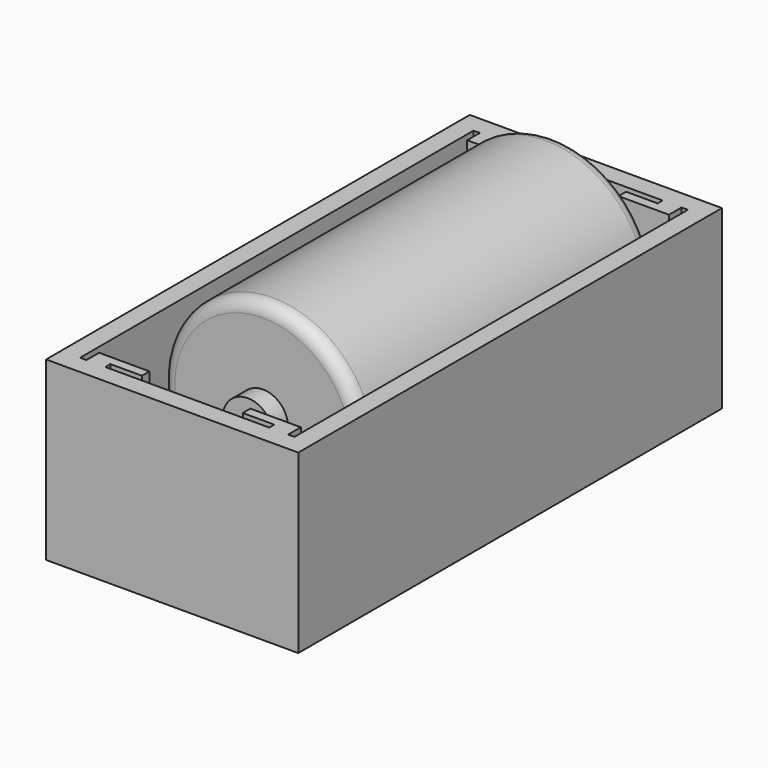
from build123d import *

# Parameters (mm, degrees)
F0_R            = 16
F1_DEPTH        = 58
F2_R            = 4
F3_DEPTH        = 3
F4_R            = 2
F6_W            = 40
F6_H            = 84
F7_DEPTH        = 3
F8_W            = 40
F8_H            = 84
F8_W_2          = 34
F8_H_2          = 78
F9_DEPTH        = 25
F10_R           = 5.8847523539
F11_DEPTH       = 25
F13_DEPTH       = 25
F14_TEXT_SIZE   = 13.9910155364
F14_TEXT_SIZE_2 = 12.9334014168
F15_DEPTH       = 0.5


# Not quite as in the source:
# - Text() gives the source's letters only with a copy of the font that has no kerning and outlines rounded to 1/6400 em; it was checked with that copy


with BuildPart() as f1:
    # F0 (on Front) → F1 (new body)
    with BuildSketch(Plane.XZ):
        Circle(F0_R)
    extrude(amount=F1_DEPTH)

    # F2 (on face) → F3 (join)
    with BuildSketch(Plane.XZ.offset(58)):
        Circle(F2_R)
    extrude(amount=F3_DEPTH)

    # F4
    f4_edges = [f1.edges().sort_by_distance(p)[0] for p in [
        (-16, -58, 0),
        (-16, 0, 0),
    ]]
    fillet(f4_edges, radius=F4_R)


with BuildPart() as f7:
    # F6 (on offset) → F7 (new body)
    with BuildSketch(Plane.XY.offset(-16)):
        with Locations((0, -34)):
            Rectangle(F6_W, F6_H)
    extrude(amount=-F7_DEPTH)

    # F8 (on face) → F9 (join)
    with BuildSketch(Plane.XY.offset(-16)):
        with Locations((0, -34)):
            Rectangle(F8_W, F8_H)
        with Locations((0, -34)):
            Rectangle(F8_W_2, F8_H_2, mode=Mode.SUBTRACT)
    extrude(amount=F9_DEPTH)

    # F10 (on face) → F11 (cut)
    with BuildSketch(Plane(origin=(0, 0, -19), x_dir=(1, 0, 0), z_dir=(0, 0, -1))):
        with Locations((-4.9920217134, 45.0053848326)):
            Circle(F10_R)
        Polygon((-6.232730113, 13.6288285578), (-6.232730113, 8.465465871), (-2.5816813434, 4.8144171014), (2.5816813434, 4.8144171014), (6.232730113, 8.465465871), (6.232730113, 13.6288285578), (2.5816813434, 17.2798773274), (-2.5816813434, 17.2798773274), align=None)
    extrude(amount=-F11_DEPTH, mode=Mode.SUBTRACT)

    # F12 (on face) → F13 (join)
    with BuildSketch(Plane.XY.offset(-16)):
        Polygon((16, 2.5), (16, 5), (13, 5), (13, 4), (8, 4), (8, 2.5), align=None)
        Polygon((-16, 2.5), (-8, 2.5), (-8, 4), (-13, 4), (-13, 5), (-16, 5), align=None)
        Polygon((-8, -72), (-8, -70.5), (-16, -70.5), (-16, -73), (-13, -73), (-13, -72), align=None)
        Polygon((13, -72), (13, -73), (16, -73), (16, -70.5), (8, -70.5), (8, -72), align=None)
    extrude(amount=F13_DEPTH)

    # F14 (on face) → F15 (cut)
    with BuildSketch(Plane(origin=(-20, 0, 0), x_dir=(0, -1, 0), z_dir=(-1, 0, 0))):
        with Locations((0.2928902395, -4.8578013666)):
            Text("Deshna's", F14_TEXT_SIZE, font='Open Sans', font_style=FontStyle.BOLD, text_align=(TextAlign.LEFT, TextAlign.BOTTOM))
        with Locations((19.8029056191, -15.7106751576)):
            Text('cell', F14_TEXT_SIZE_2, font='Open Sans', font_style=FontStyle.BOLD, text_align=(TextAlign.LEFT, TextAlign.BOTTOM))
    extrude(amount=-F15_DEPTH, mode=Mode.SUBTRACT)


solid = Compound([f1.part, f7.part])
